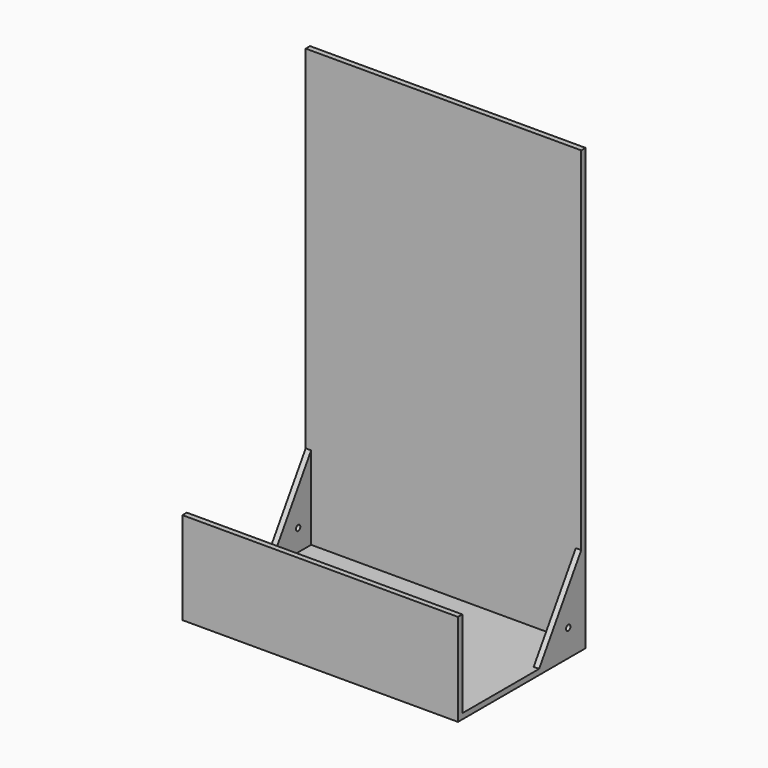
from build123d import *

# Parameters (mm, degrees)
F0_W     = 482.6
F0_H     = 279.4
F1_DEPTH = 4.7625
F2_W     = 482.6
F2_H     = 762
F3_DEPTH = 9.525
F4_W     = 482.6
F4_H     = 152.4
F5_DEPTH = 9.525
F7_DEPTH = 9.525
F9_D     = 9.525


# Not quite as in the source:
# - a pattern or mirror of a feature is missing from the dataset's text; its kind, count and spacing are read off the source's solid


with BuildPart() as f1:
    # F0 (on Top) → F1 (new body, symmetric)
    with BuildSketch(Plane.XY):
        Rectangle(F0_W, F0_H)
    extrude(amount=F1_DEPTH, both=True)

    # F2 (on face) → F3 (join)
    with BuildSketch(Plane(origin=(0, 139.7, 0), x_dir=(-1, 0, 0), z_dir=(0, 1, 0))):
        with Locations((0, 385.7625)):
            Rectangle(F2_W, F2_H)
    extrude(amount=-F3_DEPTH)

    # F4 (on face) → F5 (join)
    with BuildSketch(Plane.XZ.offset(139.7)):
        with Locations((0, 80.9625)):
            Rectangle(F4_W, F4_H)
    extrude(amount=-F5_DEPTH)

    # F6 (on face) → F7 (join)
    with BuildSketch(Plane(origin=(-241.3, 0, 0), x_dir=(0, -1, 0), z_dir=(-1, 0, 0))):
        Polygon((-37.9520058632, 4.7625), (-130.175, 150.3834724426), (-130.175, 4.7625), align=None)
    f7 = extrude(amount=-F7_DEPTH)

    # F7_copies: F7 across plane
    add(f7.mirror(Plane(origin=(0, 0, 0), x_dir=(0, 0, 1), z_dir=(1, 0, 0))))

    # F9 (through all)
    with Locations(Plane.YZ.offset(241.3)):
        with Locations((101.7590165138, 42.3114337027)):
            Hole(F9_D / 2)


solid = f1.part
